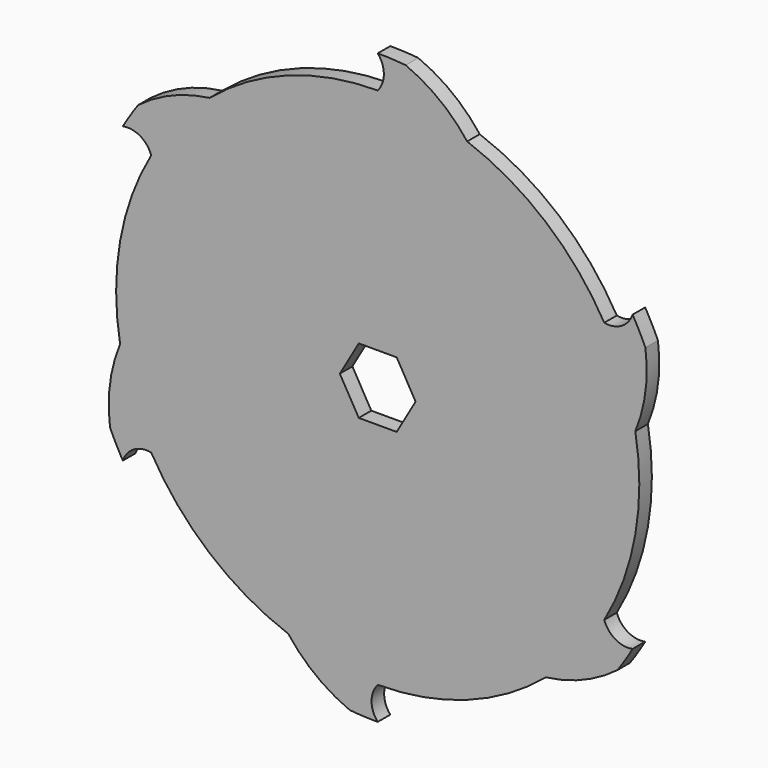
from build123d import *

# Parameters (mm, degrees)
F0_R            = 50.00625
F1_DEPTH        = 1.3335
F3_DEPTH        = 25.4
F3_DEPTH_BACK   = 25.4
F3_COPIES_COUNT = 6


# Not quite as in the source:
# - a pattern or mirror of a feature is missing from the dataset's text; its kind, count and spacing are read off the source's solid


with BuildPart() as f1:
    # F0 (on Front) → F1 (new body, symmetric)
    with BuildSketch(Plane.XZ):
        Circle(F0_R)
        Polygon((-6.4378019116, 0), (-3.2189009558, 5.5753), (3.2189009558, 5.5753), (6.4378019116, 0), (3.2189009558, -5.5753), (-3.2189009558, -5.5753), align=None, mode=Mode.SUBTRACT)
    extrude(amount=F1_DEPTH, both=True)

    # F2 (on Front) → F3 (cut, two sides)
    with BuildSketch(Plane.XZ) as f3_sk:
        with BuildLine():
            ThreePointArc((-28.5719092506, 34.0506754966), (-15.2027953708, 41.7693369939), (0, 44.45))
            ThreePointArc((0, 44.45), (1.0438391194, 47.228125), (0, 50.00625))
            ThreePointArc((0, 50.00625), (-22.9125377043, 44.4481794342), (-40.7317320204, 29.0094992318))
            ThreePointArc((-40.7317320204, 29.0094992318), (-34.9840642297, 32.3314922368), (-28.5719092506, 34.0506754966))
        make_face()
    f3 = extrude(amount=-F3_DEPTH, mode=Mode.SUBTRACT) + extrude(f3_sk.sketch, amount=F3_DEPTH_BACK, mode=Mode.SUBTRACT)

    # F3_copies: F3 ×6 about axis
    f3_copies_axis = Axis((0, 0, 0), (0, 1, 0))
    for i in range(1, F3_COPIES_COUNT):
        add(f3.rotate(f3_copies_axis, i * 360 / F3_COPIES_COUNT), mode=Mode.SUBTRACT)


solid = f1.part
